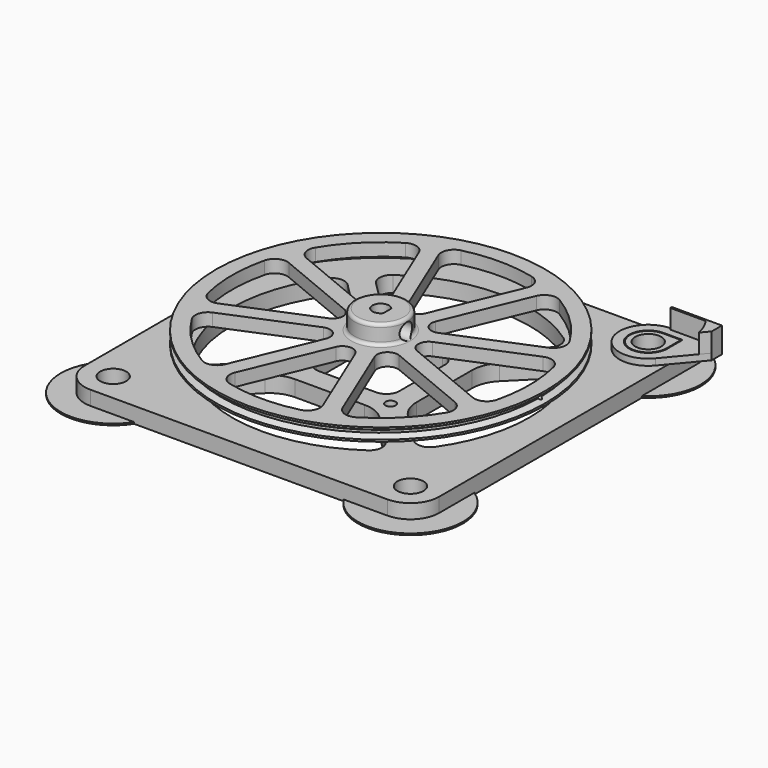
from build123d import *

# Parameters (mm, degrees)
F0_R            = 51.75
F1_DEPTH        = 4
F6_DEPTH        = 12.5
F6_COPIES_COUNT = 8
F7_DEPTH        = 12.5
F8_R            = 8.25
F9_DEPTH        = 6
F10_R           = 1
F11_R           = 2.45
F12_DEPTH       = 25
F14_R           = 0.75
F15_REACH       = 105.6223203436
F17_R           = 4.1
F17_R_2         = 2.8
F18_DEPTH       = 5
F19_R           = 1.6
F20_DEPTH       = 25
F21_R           = 1.6
F21_W           = 26.0502525317
F21_H           = 26.0502525317
F22_DEPTH       = 5.001
F23_R           = 4.1
F24_DEPTH       = 2
F25_R           = 16.5
F25_R_2         = 4.1
F26_DEPTH       = 0.5
F27_R           = 4
F28_R           = 10
F30_DEPTH       = 2
F33_DEPTH       = 6


# Not quite as in the source:
# - a pattern or mirror of a feature is missing from the dataset's text; its kind, count and spacing are read off the source's solid


with BuildPart() as f1:
    # F0 (on Top) → F1 (new body)
    with BuildSketch(Plane.XY):
        Circle(F0_R)
    extrude(amount=F1_DEPTH)

    # F2 (on Front) → F3 (revolve, cut)
    with BuildSketch(Plane.XZ):
        Polygon((51.75, 0.6), (51.75, 3.4), (50, 2.3896370289), (50, 1.6103629711), align=None)
    revolve(axis=Axis((0, 0, 4), (0, 0, 1)), mode=Mode.SUBTRACT)

    # F5 (on face) → F6 (cut, symmetric)
    with BuildSketch(Plane.XY.offset(4)):
        with BuildLine():
            Line((39.9933521052, 13.859808346), (13.8472470688, 3.0297370367))
            ThreePointArc((13.8472470688, 3.0297370367), (11.8228415024, 0), (13.8472470688, -3.0297370367))
            Line((13.8472470688, -3.0297370367), (39.9933521052, -13.859808346))
            ThreePointArc((39.9933521052, -13.859808346), (43.3321297514, -13.7323397104), (45.4093804157, -11.1153349145))
            ThreePointArc((45.4093804157, -11.1153349145), (46.75, 0), (45.4093804157, 11.1153349145))
            ThreePointArc((45.4093804157, 11.1153349145), (43.3321297514, 13.7323397104), (39.9933521052, 13.859808346))
        make_face()
    f6 = extrude(amount=F6_DEPTH, both=True, mode=Mode.SUBTRACT)

    # F6_copies: F6 ×8 about axis
    f6_copies_axis = Axis((0, 0, 0), (0, 0, 1))
    for i in range(1, F6_COPIES_COUNT):
        add(f6.rotate(f6_copies_axis, i * 360 / F6_COPIES_COUNT), mode=Mode.SUBTRACT)

    # F4 (on Top) → F7 (cut, symmetric)
    with BuildSketch(Plane.XY):
        with BuildLine():
            Line((2.09, -1.5465768652), (2.09, 1.5465768652))
            ThreePointArc((2.09, 1.5465768652), (-2.6, 0), (2.09, -1.5465768652))
        make_face()
    extrude(amount=F7_DEPTH, both=True, mode=Mode.SUBTRACT)

    # F8 (on face) → F9 (join)
    with BuildSketch(Plane.XY.offset(4)):
        Circle(F8_R)
        with BuildLine():
            ThreePointArc((2.09, -1.5465768652), (-2.6, 0), (2.09, 1.5465768652))
            Line((2.09, 1.5465768652), (2.09, -1.5465768652))
        make_face(mode=Mode.SUBTRACT)
    extrude(amount=F9_DEPTH)

    # F10
    f10_edges = [f1.edges().sort_by_distance(p)[0] for p in [
        (-8.25, 0, 4),
        (-8.25, 0, 10),
    ]]
    fillet(f10_edges, radius=F10_R)

    # F11 (on Right) → F12 (cut)
    with BuildSketch(Plane.YZ):
        with Locations((0, 6.45)):
            Circle(F11_R)
    extrude(amount=F12_DEPTH, mode=Mode.SUBTRACT)

    f15_end = f1.faces().sort_by_distance((46.75, 0, 2))[0]
    # F14 (on plane+point) → F15 (cut, up to a face of the model that its end follows)
    with BuildSketch(Plane.YZ.offset(51.75)):
        with Locations((0, 2)):
            Circle(F14_R)
    f15_long = extrude(amount=-F15_REACH, mode=Mode.PRIVATE)
    add(split(f15_long, bisect_by=f15_end, keep=Keep.BOTTOM, mode=Mode.PRIVATE), mode=Mode.SUBTRACT)


with BuildPart() as f18:
    # F17 (on offset) → F18 (new body)
    with BuildSketch(Plane.XY.offset(-5)):
        with BuildLine():
            Line((46.73, 55.75), (0, 55.75))
            ThreePointArc((0, 55.75), (39.4212030512, 39.4212030512), (55.75, 0))
            Line((55.75, 0), (55.75, 55.75))
            Line((55.75, 55.75), (46.73, 55.75))
        make_face()
        with Locations((46.73, 46.73)):
            Circle(F17_R, mode=Mode.SUBTRACT)
        with BuildLine():
            ThreePointArc((55.75, 0), (39.4212030512, 39.4212030512), (0, 55.75))
            ThreePointArc((0, 55.75), (-39.4212030512, 39.4212030512), (-55.75, 0))
            ThreePointArc((-55.75, 0), (-39.4212031068, -39.4212029955), (-1.575e-07, -55.75))
            ThreePointArc((-1.575e-07, -55.75), (39.4212029955, -39.4212031068), (55.75, 0))
        make_face()
        Circle(F17_R_2, mode=Mode.SUBTRACT)
        with BuildLine():
            Line((55.75, -46.73), (55.75, 0))
            ThreePointArc((55.75, 0), (39.4212029955, -39.4212031068), (-1.575e-07, -55.75))
            Line((-1.575e-07, -55.75), (46.73, -55.75))
            ThreePointArc((46.73, -55.75), (53.1081031663, -53.1081031663), (55.75, -46.73))
        make_face()
        with Locations((46.73, -46.73)):
            Circle(F17_R, mode=Mode.SUBTRACT)
        with BuildLine():
            ThreePointArc((-1.575e-07, -55.75), (-39.4212031068, -39.4212029955), (-55.75, 0))
            Line((-55.75, 0), (-55.75, -46.73))
            ThreePointArc((-55.75, -46.73), (-53.1081031663, -53.1081031663), (-46.73, -55.75))
            Line((-46.73, -55.75), (-1.575e-07, -55.75))
        make_face()
        with Locations((-46.73, -46.73)):
            Circle(F17_R, mode=Mode.SUBTRACT)
    extrude(amount=-F18_DEPTH)

    # F19 (on face) → F20 (cut)
    with BuildSketch(Plane.XY.offset(-5)):
        with Locations((-15.5, 15.5)):
            Circle(F19_R)
        with Locations((15.5, -15.5)):
            Circle(F19_R)
        with Locations((15.5, 15.5)):
            Circle(F19_R)
        with Locations((-15.5, -15.5)):
            Circle(F19_R)
    extrude(amount=-F20_DEPTH, mode=Mode.SUBTRACT)

    # F21 (on face) → F22 (cut, through all)
    with BuildSketch(Plane.XY.offset(-5)):
        with BuildLine():
            Line((-20.0251262658, -15.0753787975), (-20.0251262658, 15.0753787975))
            Line((-20.0251262658, 15.0753787975), (-35.439343243, 30.4895957747))
            ThreePointArc((-35.439343243, 30.4895957747), (-46.75, 0), (-35.439343243, -30.4895957747))
            Line((-35.439343243, -30.4895957747), (-20.0251262658, -15.0753787975))
        make_face()
        with BuildLine():
            Line((-30.4895957747, 35.439343243), (-15.0753787975, 20.0251262658))
            Line((-15.0753787975, 20.0251262658), (15.0753787975, 20.0251262658))
            Line((15.0753787975, 20.0251262658), (30.4895957747, 35.439343243))
            ThreePointArc((30.4895957747, 35.439343243), (0, 46.75), (-30.4895957747, 35.439343243))
        make_face()
        with BuildLine():
            Line((35.439343243, 30.4895957747), (20.0251262658, 15.0753787975))
            Line((20.0251262658, 15.0753787975), (20.0251262658, -15.0753787975))
            Line((20.0251262658, -15.0753787975), (35.439343243, -30.4895957747))
            ThreePointArc((35.439343243, -30.4895957747), (46.75, 0), (35.439343243, 30.4895957747))
        make_face()
        with BuildLine():
            Line((30.4895957747, -35.439343243), (15.0753787975, -20.0251262658))
            Line((15.0753787975, -20.0251262658), (-15.0753787975, -20.0251262658))
            Line((-15.0753787975, -20.0251262658), (-30.4895957747, -35.439343243))
            ThreePointArc((-30.4895957747, -35.439343243), (0, -46.75), (30.4895957747, -35.439343243))
        make_face()
        with Locations((-15.5, 15.5)):
            Circle(F21_R)
        with Locations((15.5, 15.5)):
            Circle(F21_R)
        with Locations((-15.5, -15.5)):
            Circle(F21_R)
        with Locations((15.5, -15.5)):
            Circle(F21_R)
        Rectangle(F21_W, F21_H)
    extrude(amount=-F22_DEPTH, mode=Mode.SUBTRACT)

    # F23 (on face) → F24 (join)
    with BuildSketch(Plane.XY.offset(-5)):
        with BuildLine():
            ThreePointArc((46.73, 52.43), (42.6994913472, 42.6994913472), (52.43, 46.73))
            ThreePointArc((52.43, 46.73), (50.7605086528, 50.7605086528), (46.73, 52.43))
        make_face()
        with Locations((46.73, 46.73)):
            Circle(F23_R, mode=Mode.SUBTRACT)
        with BuildLine():
            ThreePointArc((46.73, 52.43), (50.7605086528, 50.7605086528), (52.43, 46.73))
            Line((52.43, 46.73), (52.43, 52.43))
            Line((52.43, 52.43), (46.73, 52.43))
        make_face()
    extrude(amount=F24_DEPTH)

    # F25 (on face) → F26 (join)
    with BuildSketch(Plane(origin=(0, 0, -10), x_dir=(1, 0, 0), z_dir=(0, 0, -1))):
        with Locations((-46.73, 46.73)):
            Circle(F25_R)
        with Locations((-46.73, 46.73)):
            Circle(F25_R_2, mode=Mode.SUBTRACT)
        with Locations((46.73, 46.73)):
            Circle(F25_R)
        with Locations((46.73, 46.73)):
            Circle(F25_R_2, mode=Mode.SUBTRACT)
        with Locations((46.73, -46.73)):
            Circle(F25_R)
        with Locations((46.73, -46.73)):
            Circle(F25_R_2, mode=Mode.SUBTRACT)
    extrude(amount=-F26_DEPTH)

    # F27
    f27_edges = [f18.edges().sort_by_distance(p)[0] for p in [
        (-35.439343, -30.489596, -7.5),
        (-30.489596, 35.439343, -7.5),
        (30.489596, 35.439343, -7.5),
        (35.439343, 30.489596, -7.5),
        (-35.439343, 30.489596, -7.5),
        (35.439343, -30.489596, -7.5),
        (30.489596, -35.439343, -7.5),
        (-30.489596, -35.439343, -7.5),
        (-13.025126, -13.025126, -7.5),
        (-13.025126, 13.025126, -7.5),
        (13.025126, -13.025126, -7.5),
        (13.025126, 13.025126, -7.5),
    ]]
    fillet(f27_edges, radius=F27_R)

    # F28
    f28_edges = [f18.edges().sort_by_distance(p)[0] for p in [
        (-15.075379, -20.025126, -7.5),
        (15.075379, -20.025126, -7.5),
        (-20.025126, 15.075379, -7.5),
        (-20.025126, -15.075379, -7.5),
        (15.075379, 20.025126, -7.5),
        (-15.075379, 20.025126, -7.5),
        (20.025126, -15.075379, -7.5),
        (20.025126, 15.075379, -7.5),
    ]]
    fillet(f28_edges, radius=F28_R)


with BuildPart() as f30:
    # F29 (on face) → F30 (new body)
    with BuildSketch(Plane.XY.offset(-5)):
        with BuildLine():
            Line((55.75, 55.75), (46.73, 55.75))
            ThreePointArc((46.73, 55.75), (38.556452792, 42.9150916081), (53.6438212495, 40.9369459065))
            ThreePointArc((53.6438212495, 40.9369459065), (55.2071182506, 43.6479769364), (55.75, 46.73))
            Line((55.75, 46.73), (55.75, 55.75))
        make_face()
        with BuildLine():
            ThreePointArc((52.73, 46.73), (42.4873593129, 42.4873593129), (46.73, 52.73))
            Line((46.73, 52.73), (52.73, 52.73))
            Line((52.73, 52.73), (52.73, 46.73))
        make_face(mode=Mode.SUBTRACT)
        with BuildLine():
            ThreePointArc((55.75, 46.73), (55.2071182506, 43.6479769364), (53.6438212495, 40.9369459065))
            Line((53.6438212495, 40.9369459065), (62.68, 51.7213307321))
            Line((62.68, 51.7213307321), (62.68, 55.75))
            Line((62.68, 55.75), (55.75, 55.75))
            Line((55.75, 55.75), (55.75, 46.73))
        make_face()
    extrude(amount=F30_DEPTH)

    # F32 (on face) → F33 (join)
    with BuildSketch(Plane.XY.offset(-3)):
        with BuildLine():
            ThreePointArc((58.0612280145, 55.1212616265), (59.6707600721, 52.3288149422), (60.6041029548, 49.2438152677))
            Line((60.6041029548, 49.2438152677), (62.68, 51.7213307321))
            Line((62.68, 51.7213307321), (62.68, 55.75))
            Line((62.68, 55.75), (58.68, 55.75))
            Line((58.68, 55.75), (58.68, 55.1212616265))
            Line((58.68, 55.1212616265), (58.0612280145, 55.1212616265))
        make_face()
        with BuildLine():
            Line((46.9631627202, 55.1212616265), (58.0612280145, 55.1212616265))
            ThreePointArc((58.0612280145, 55.1212616265), (57.8187794518, 55.4391314302), (57.5674166663, 55.75))
            Line((57.5674166663, 55.75), (46.9631627202, 55.75))
            Line((46.9631627202, 55.75), (46.9631627202, 55.1212616265))
        make_face()
        with BuildLine():
            ThreePointArc((57.5674166663, 55.75), (57.8187794518, 55.4391314302), (58.0612280145, 55.1212616265))
            Line((58.0612280145, 55.1212616265), (58.68, 55.1212616265))
            Line((58.68, 55.1212616265), (58.68, 55.75))
            Line((58.68, 55.75), (57.5674166663, 55.75))
        make_face()
    extrude(amount=F33_DEPTH)


solid = Compound([f1.part, f18.part, f30.part])
